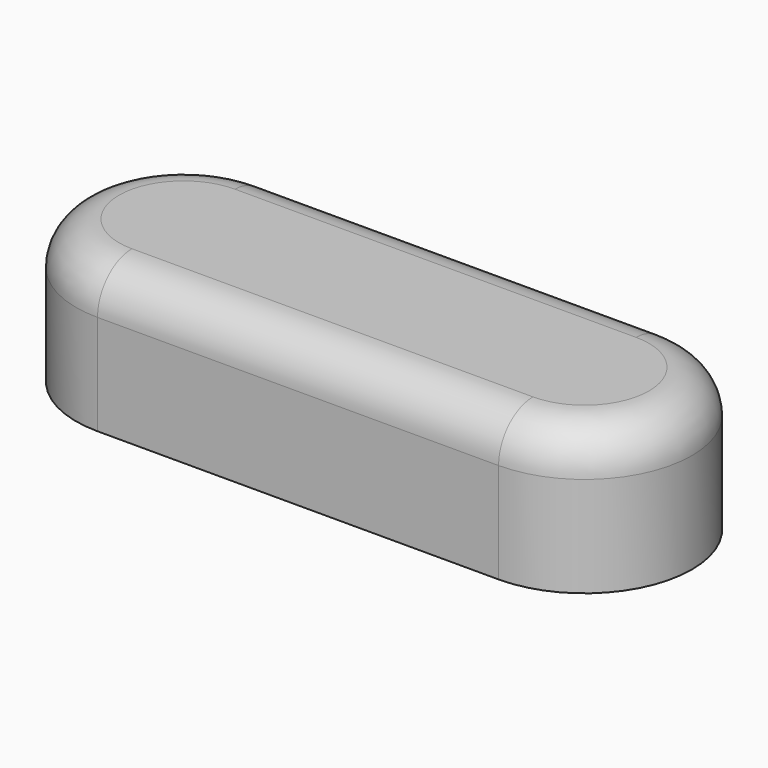
from build123d import *

# Parameters (mm, degrees)
F0_W     = 63.7512656803
F0_H     = 75
F0_W_2   = 76.2487343197
F1_DEPTH = 65
F2_R     = 15
F3_T     = 2.5


# Not quite as in the source:
# - a shell that OpenCascade refuses in one call is made with other operations: the cavity is built on its own and cut out


with BuildPart() as f1:
    # F0 (on Top) → F1 (new body)
    with BuildSketch(Plane.XY):
        with BuildLine():
            Line((-63.7512656803, -75), (-63.7512656803, 0))
            ThreePointArc((-63.7512656803, 0), (-101.2512656803, -37.5), (-63.7512656803, -75))
        make_face()
        with Locations((-31.8756328402, -37.5)):
            Rectangle(F0_W, F0_H)
        with Locations((38.1243671598, -37.5)):
            Rectangle(F0_W_2, F0_H)
        with BuildLine():
            ThreePointArc((76.2487343197, -75), (113.7487343197, -37.5), (76.2487343197, 0))
            Line((76.2487343197, 0), (76.2487343197, -75))
        make_face()
    extrude(amount=F1_DEPTH)

    # F2
    f2_edges = [f1.edges().sort_by_distance(p)[0] for p in [
        (-101.251266, -37.5, 65),
        (113.748734, -37.5, 0),
        (6.248734, -75, 65),
        (113.748734, -37.5, 65),
        (6.248734, 0, 65),
    ]]
    fillet(f2_edges, radius=F2_R)

    # F3: shell of thickness 2.5, made by hand


with BuildPart() as f3_core1:
    # F3_t2: copy of F1
    add(f1.part)

    # the walls: a layer under each face that stays
    f3_faces = [f3_core1.faces().sort_by_distance(p)[0] for p in [
        (-101.2512656803, -37.5, 32.5),
        (6.2487343197, 0, 32.5),
        (-96.8578673981, -37.5, 60.6066017178),
        (6.2487343197, -75, 32.5),
        (113.7487343197, -37.5, 32.5),
        (6.2487343197, -4.3933982822, 60.6066017178),
        (6.2487343197, -37.5, 65),
        (6.2487343197, -70.6066017178, 60.6066017178),
        (109.3553360375, -37.5, 60.6066017178),
    ]]
    thicken(f3_faces, amount=-F3_T, mode=Mode.SUBTRACT)


with BuildPart() as f1_1:
    add(f1.part)

    # what is left inside the walls is the cavity
    f3_cavity = [f3_core1.part.solids().sort_by_distance(p)[0] for p in [
        (6.248734, -45, 0.025),
    ]]
    add(f3_cavity, mode=Mode.SUBTRACT)


solid = f1_1.part
